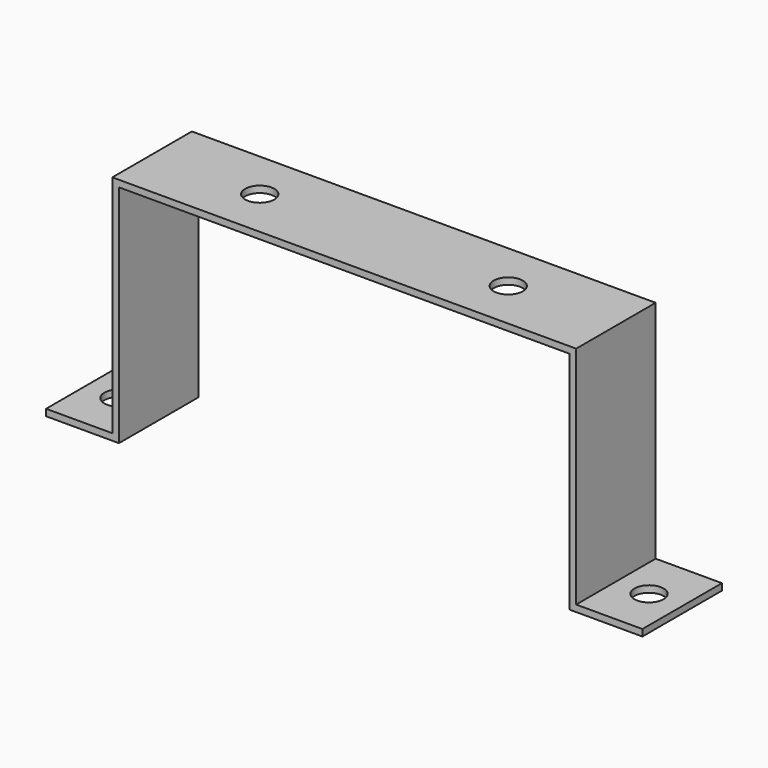
from build123d import *

# Parameters (mm, degrees)
F1_DEPTH = 30
F2_R     = 4.4
F3_R     = 4.4
F4_DEPTH = 25


# Not quite as in the source:
# - a feature names something its author has since deleted; it is built from what else it names


with BuildPart() as f1:
    # F0 (on Front) → F1 (new body)
    with BuildSketch(Plane.XZ):
        Polygon((90, -1), (90, 1), (70, 1), (70, 69), (-70, 69), (-70, 1), (-90, 1), (-90, -1), (-68, -1), (-68, 67), (68, 67), (68, -1), align=None)
    extrude(amount=F1_DEPTH)

    # F2 (on face) + F3 (on face) → F4 (cut)
    with BuildSketch(Plane.XY.offset(1)):
        with Locations((-80, -15)):
            Circle(F2_R)
        with Locations((80, -15)):
            Circle(F2_R)
    with BuildSketch(Plane.XY.offset(69)):
        with Locations((-37.5, -15)):
            Circle(F3_R)
        with Locations((37.5, -15)):
            Circle(F3_R)
    extrude(amount=-F4_DEPTH, mode=Mode.SUBTRACT)


solid = f1.part
